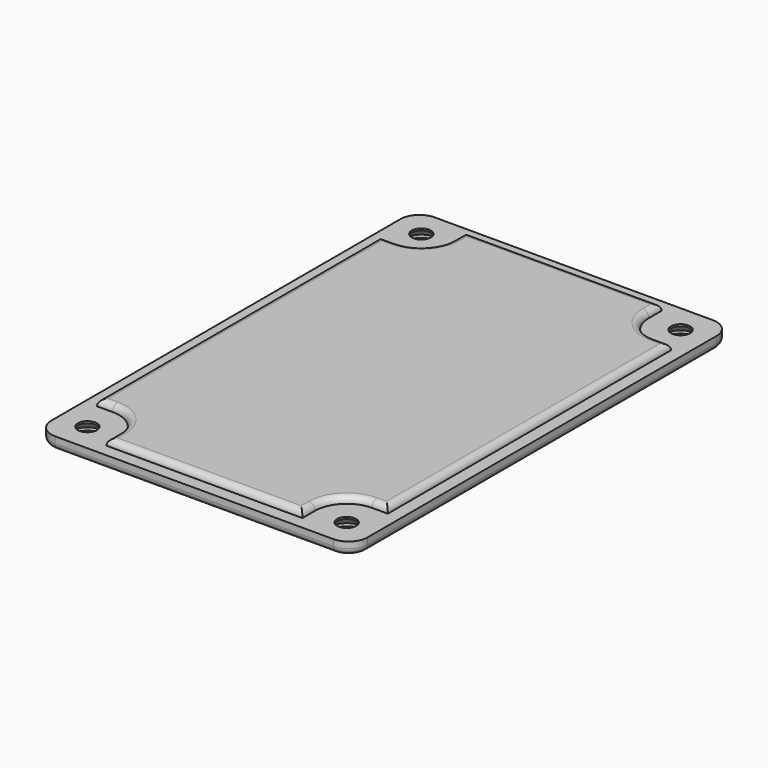
from build123d import *

# Parameters (mm, degrees)
F1_DEPTH  = 2
F2_R      = 1.5
F3_DEPTH  = 5
F4_W      = 31
F4_H      = 56
F5_DEPTH  = 1
F6_R      = 0.99999
F7_R      = 1
F8_R      = 2.8
F9_DEPTH  = 0.5
F10_SIZE2 = 1.2
F10_SIZE  = 1.2


# Not quite as in the source:
# - a fillet or chamfer is up to 0.001 mm smaller than in the source, because OpenCascade refuses the exact size
# - a feature names something its author has since deleted; it is built from what else it names


with BuildPart() as f1:
    # F0 (on Top) → F1 (new body)
    with BuildSketch(Plane.XY):
        with BuildLine():
            ThreePointArc((0, 3), (0.8786796564, 0.8786796564), (3, 0))
            Line((3, 0), (47, 0))
            ThreePointArc((47, 0), (49.1213203436, 0.8786796564), (50, 3))
            Line((50, 3), (50, 72))
            ThreePointArc((50, 72), (49.1213203436, 74.1213203436), (47, 75))
            Line((47, 75), (3, 75))
            ThreePointArc((3, 75), (0.8786796564, 74.1213203436), (0, 72))
            Line((0, 72), (0, 3))
        make_face()
    extrude(amount=F1_DEPTH)

    # F2 (on face) → F3 (cut)
    with BuildSketch(Plane.XY.offset(2)):
        with Locations((4.5, 70.5)):
            Circle(F2_R)
        with Locations((45.5, 70.5)):
            Circle(F2_R)
        with Locations((4.5, 4.5)):
            Circle(F2_R)
        with Locations((45.5, 4.5)):
            Circle(F2_R)
    extrude(amount=-F3_DEPTH, mode=Mode.SUBTRACT)

    # F4 (on face) → F5 (join)
    with BuildSketch(Plane.XY.offset(2)):
        Polygon((9.5, 9.5), (9.5, 4.5), (9.5, 2), (40.5, 2), (40.5, 4.5), (40.5, 9.5), align=None)
        Polygon((9.5, 70.5), (9.5, 65.5), (40.5, 65.5), (40.5, 70.5), (40.5, 73), (9.5, 73), align=None)
        Polygon((2, 9.5), (4.5, 9.5), (9.5, 9.5), (9.5, 65.5), (4.5, 65.5), (2, 65.5), align=None)
        with Locations((25, 37.5)):
            Rectangle(F4_W, F4_H)
        Polygon((40.5, 65.5), (40.5, 9.5), (45.5, 9.5), (48, 9.5), (48, 65.5), (45.5, 65.5), align=None)
        with BuildLine():
            Line((4.5, 65.5), (9.5, 65.5))
            Line((9.5, 65.5), (9.5, 70.5))
            ThreePointArc((9.5, 70.5), (8.0355339059, 66.9644660941), (4.5, 65.5))
        make_face()
        with BuildLine():
            Line((40.5, 70.5), (40.5, 65.5))
            Line((40.5, 65.5), (45.5, 65.5))
            ThreePointArc((45.5, 65.5), (41.9644660941, 66.9644660941), (40.5, 70.5))
        make_face()
        with BuildLine():
            Line((45.5, 9.5), (40.5, 9.5))
            Line((40.5, 9.5), (40.5, 4.5))
            ThreePointArc((40.5, 4.5), (41.9644660941, 8.0355339059), (45.5, 9.5))
        make_face()
        with BuildLine():
            ThreePointArc((4.5, 9.5), (8.0355339059, 8.0355339059), (9.5, 4.5))
            Line((9.5, 4.5), (9.5, 9.5))
            Line((9.5, 9.5), (4.5, 9.5))
        make_face()
    extrude(amount=F5_DEPTH)

    # F6 (radius 1 in the source; OpenCascade refuses exactly that, so slightly less here)
    f6_edges = [f1.edges().sort_by_distance(p)[0] for p in [
        (9.5, 3.25, 3),
        (25, 2, 3),
        (40.5, 3.25, 3),
        (41.964466, 8.035534, 3),
        (46.75, 9.5, 3),
        (48, 37.5, 3),
        (46.75, 65.5, 3),
        (41.964466, 66.964466, 3),
        (40.5, 71.75, 3),
        (25, 73, 3),
        (9.5, 71.75, 3),
        (8.035534, 66.964466, 3),
        (3.25, 65.5, 3),
        (2, 37.5, 3),
        (3.25, 9.5, 3),
        (8.035534, 8.035534, 3),
    ]]
    fillet(f6_edges, radius=F6_R)

    # F7
    f7_edges = [f1.edges().sort_by_distance(p)[0] for p in [
        (0, 37.5, 0),
    ]]
    fillet(f7_edges, radius=F7_R)

    # F8 (on face) → F9 (cut)
    with BuildSketch(Plane(origin=(0, 0, 0), x_dir=(1, 0, 0), z_dir=(0, 0, -1))):
        with Locations((4.5, -4.5)):
            Circle(F8_R)
        with Locations((45.5, -4.5)):
            Circle(F8_R)
        with Locations((45.5, -70.5)):
            Circle(F8_R)
        with Locations((4.5, -70.5)):
            Circle(F8_R)
    extrude(amount=-F9_DEPTH, mode=Mode.SUBTRACT)

    # F10
    f10_edges = [f1.edges().sort_by_distance(p)[0] for p in [
        (3, 4.5, 0.5),
        (44, 4.5, 0.5),
        (3, 70.5, 0.5),
        (44, 70.5, 0.5),
    ]]
    chamfer(f10_edges, length=F10_SIZE, length2=F10_SIZE2)


solid = f1.part
